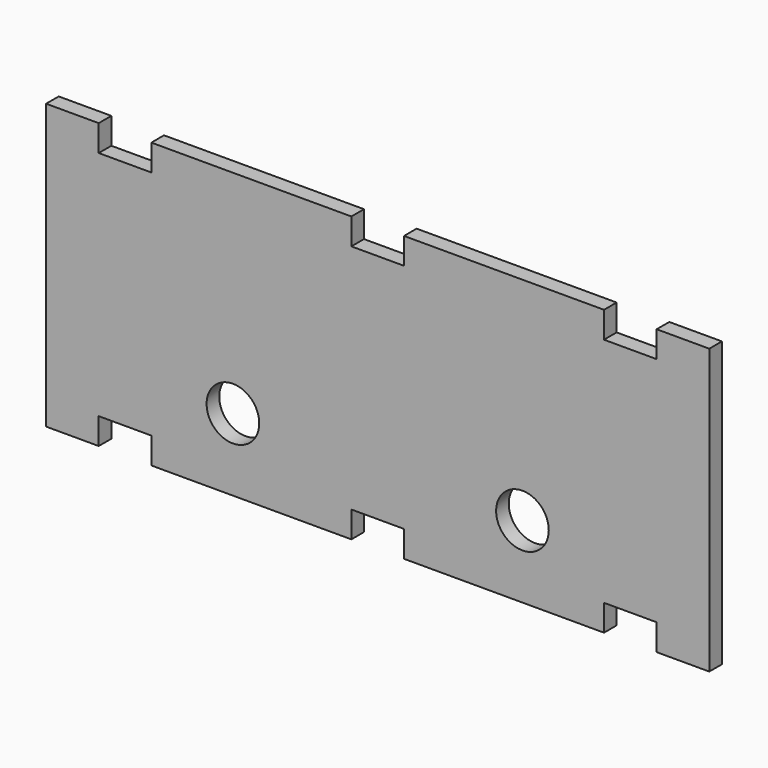
from build123d import *

# Parameters (mm, degrees)
F0_R     = 6.35
F1_DEPTH = 3.81


# Not quite as in the source:
# - a feature names something its author has since deleted; it is built from what else it names


with BuildPart() as f1:
    # F0 (on Front) → F1 (new body)
    with BuildSketch(Plane.XZ):
        Polygon((-80, 34.29), (-80, -34.29), (-67.3, -34.29), (-67.3, -27.94), (-54.6, -27.94), (-54.6, -34.29), (-6.35, -34.29), (-6.35, -27.94), (6.35, -27.94), (6.35, -34.29), (54.6, -34.29), (54.6, -27.94), (67.3, -27.94), (67.3, -34.29), (80, -34.29), (80, 34.29), (67.3, 34.29), (67.3, 27.94), (54.6, 27.94), (54.6, 34.29), (6.35, 34.29), (6.35, 27.94), (-6.35, 27.94), (-6.35, 34.29), (-54.6, 34.29), (-54.6, 27.94), (-67.3, 27.94), (-67.3, 34.29), align=None)
        with Locations((-34.925, -16.8712735176)):
            Circle(F0_R, mode=Mode.SUBTRACT)
        with Locations((34.925, -16.8712735176)):
            Circle(F0_R, mode=Mode.SUBTRACT)
    extrude(amount=F1_DEPTH)


solid = f1.part
